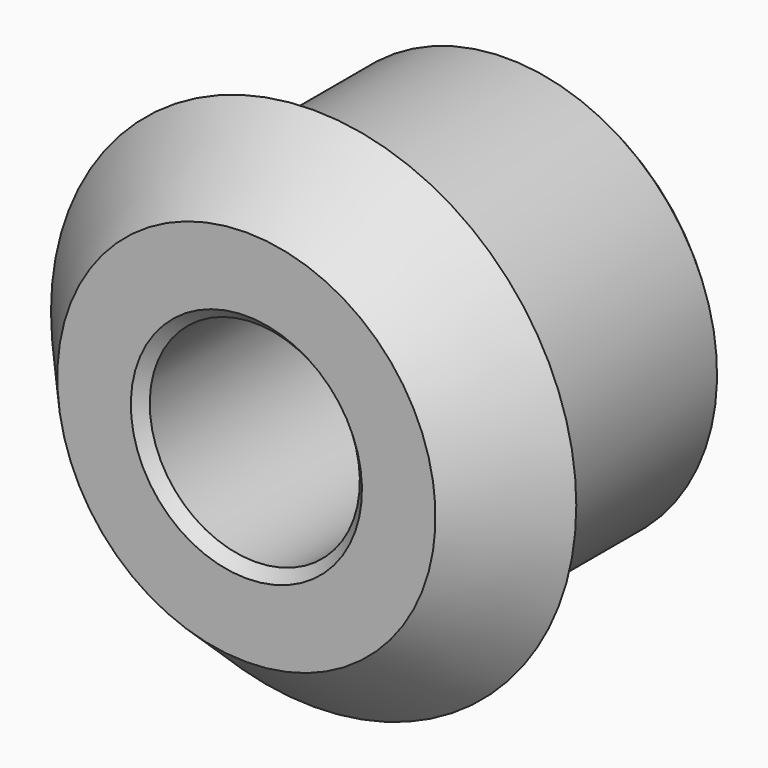
from build123d import *


# Not quite as in the source:
# - a fillet or chamfer that OpenCascade refuses, or shapes differently, is made with other operations: its cross-section is extruded or revolved along the edge and cut away or added


with BuildPart() as f1:
    # F0 (on Right) → F1 (revolve)
    with BuildSketch(Plane.YZ):
        Polygon((0, -5), (0, -2.5), (-8, -2.5), (-8, -4.5), (-6, -6.25), (-5, -5), align=None)
    revolve(axis=Axis((0, -4, 0), (0, -1, 0)))

    # F2: chamfer of 0.25 on 4 edges, made by hand

    # F2_s1 → F2_t2 (revolve)
    with BuildSketch(Plane.YZ):
        Polygon((-5.0750609905, -5.0938262381), (-4.8798437881, -5), (-5, -5), align=None)
    revolve(axis=Axis((0, -5, 0), (0, -1, 0)))

    # F2_s3 → F2_t4 (revolve, cut)
    with BuildSketch(Plane.YZ):
        Polygon((-7.75, -2.5), (-8, -2.75), (-8, -2.5), align=None)
    revolve(axis=Axis((0, -8, 0), (0, -1, 0)), mode=Mode.SUBTRACT)

    # F2_s5 → F2_t6 (revolve, cut)
    with BuildSketch(Plane.YZ):
        Polygon((0, -2.75), (-0.25, -2.5), (0, -2.5), align=None)
    revolve(axis=Axis((0, 0, 0), (0, -1, 0)), mode=Mode.SUBTRACT)

    # F2_s7 → F2_t8 (revolve, cut)
    with BuildSketch(Plane.YZ):
        Polygon((0, -4.75), (-0.25, -5), (0, -5), align=None)
    revolve(axis=Axis((0, 0, 0), (0, -1, 0)), mode=Mode.SUBTRACT)


solid = f1.part
